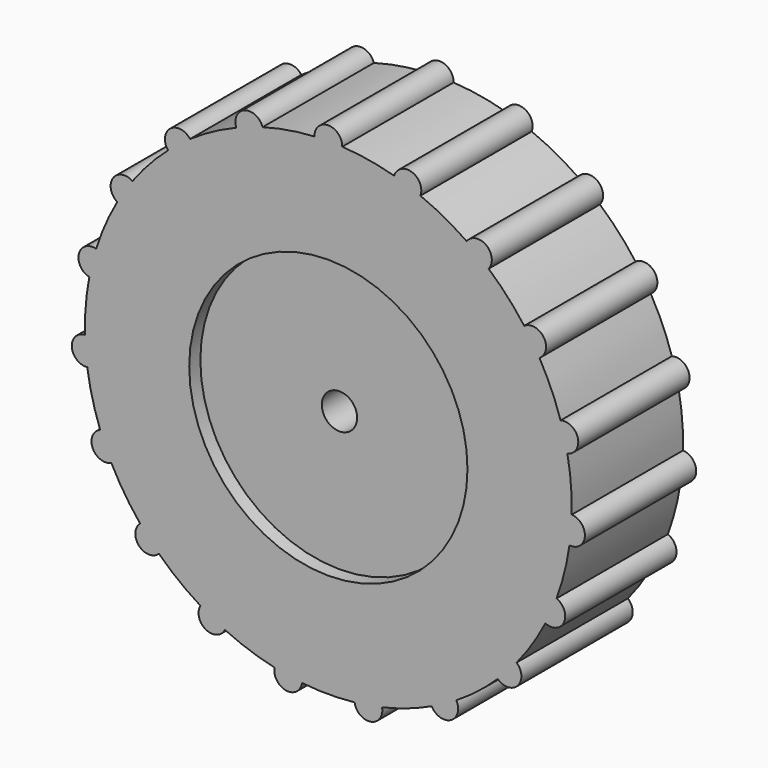
from build123d import *

# Parameters (mm, degrees)
F0_R     = 16.51
F0_R_2   = 1.6129
F1_DEPTH = 12.7
F3_R     = 12.7
F3_R_2   = 1.6129
F2_R     = 12.7
F2_R_2   = 1.6129
F4_DEPTH = 1.27
F5_DEPTH = 1.27


# Not quite as in the source:
# - the program builds the solid bodies; features that only make, move or delete a surface that nothing else refers to are left out


with BuildPart() as f1:
    # F0 (on Front) → F1 (new body)
    with BuildSketch(Plane.XZ):
        with BuildLine():
            ThreePointArc((1.2694815268, 22.1887142857), (0, 23.495), (-1.2694815268, 22.1887142857))
            ThreePointArc((-1.2694815268, 22.1887142857), (-3.658114769, 21.9218799681), (-6.0039662348, 21.3986685205))
            ThreePointArc((-6.0039662348, 21.3986685205), (-7.628814029, 22.2219760938), (-8.405361267, 20.5742685647))
            ThreePointArc((-8.405361267, 20.5742685647), (-10.5779308102, 19.5463041206), (-12.6267910938, 18.2897449866))
            ThreePointArc((-12.6267910938, 18.2897449866), (-13.6508775395, 17.5386478213), (-14.6303896913, 16.730281602))
            ThreePointArc((-14.6303896913, 16.730281602), (-16.3514639147, 15.0525829294), (-17.8813072129, 13.1988437887))
            ThreePointArc((-17.8813072129, 13.1988437887), (-18.6060249794, 12.1559228143), (-19.2699883786, 11.0733090306))
            ThreePointArc((-19.2699883786, 11.0733090306), (-20.3530621849, 8.9276808129), (-21.1981062384, 6.6776430652))
            ThreePointArc((-21.1981062384, 6.6776430652), (-21.5449209105, 5.4559149517), (-21.8213848205, 4.2163716058))
            ThreePointArc((-21.8213848205, 4.2163716058), (-22.1490903571, 1.8353259531), (-22.2177615305, -0.5671838988))
            ThreePointArc((-22.2177615305, -0.5671838988), (-22.1490903571, -1.8353259531), (-22.0080956233, -3.0974751064))
            ThreePointArc((-22.0080956233, -3.0974751064), (-21.5449209105, -5.4559149517), (-20.8297776166, -7.7505476866))
            ThreePointArc((-20.8297776166, -7.7505476866), (-20.3530621849, -8.9276808129), (-19.8098877746, -10.0756623284))
            ThreePointArc((-19.8098877746, -10.0756623284), (-18.6060249794, -12.1559228143), (-17.1845640907, -14.0940193703))
            ThreePointArc((-17.1845640907, -14.0940193703), (-16.3514639147, -15.0525829294), (-15.4649712035, -15.9619951972))
            ThreePointArc((-15.4649712035, -15.9619951972), (-13.6508775395, -17.5386478213), (-11.6771363996, -18.9101853641))
            ThreePointArc((-11.6771363996, -18.9101853641), (-10.5779308102, -19.5463041206), (-9.4441850386, -20.1185982105))
            ThreePointArc((-9.4441850386, -20.1185982105), (-7.2164457031, -21.0207881968), (-4.9043097902, -21.6771393519))
            ThreePointArc((-4.9043097902, -21.6771393519), (-3.658114769, -21.9218799681), (-2.3999748833, -22.0950389355))
            ThreePointArc((-2.3999748833, -22.0950389355), (0, -22.225), (2.3999748833, -22.0950389355))
            ThreePointArc((2.3999748833, -22.0950389355), (3.658114769, -21.9218799681), (4.9043097902, -21.6771393519))
            ThreePointArc((4.9043097902, -21.6771393519), (7.2164457031, -21.0207881968), (9.4441850386, -20.1185982105))
            ThreePointArc((9.4441850386, -20.1185982105), (10.5779308102, -19.5463041206), (11.6771363996, -18.9101853641))
            ThreePointArc((11.6771363996, -18.9101853641), (13.6508775395, -17.5386478213), (15.4649712035, -15.9619951972))
            ThreePointArc((15.4649712035, -15.9619951972), (16.3514639147, -15.0525829294), (17.1845640907, -14.0940193703))
            ThreePointArc((17.1845640907, -14.0940193703), (18.6060249794, -12.1559228143), (19.8098877746, -10.0756623284))
            ThreePointArc((19.8098877746, -10.0756623284), (20.3530621849, -8.9276808129), (20.8297776166, -7.7505476866))
            ThreePointArc((20.8297776166, -7.7505476866), (21.5449209105, -5.4559149517), (22.0080956233, -3.0974751064))
            ThreePointArc((22.0080956233, -3.0974751064), (22.1490903571, -1.8353259531), (22.2177615305, -0.5671838988))
            ThreePointArc((22.2177615305, -0.5671838988), (22.1490903571, 1.8353259531), (21.8213848205, 4.2163716058))
            ThreePointArc((21.8213848205, 4.2163716058), (21.5449209105, 5.4559149517), (21.1981062384, 6.6776430652))
            ThreePointArc((21.1981062384, 6.6776430652), (20.3530621849, 8.9276808129), (19.2699883786, 11.0733090306))
            ThreePointArc((19.2699883786, 11.0733090306), (18.6060249794, 12.1559228143), (17.8813072129, 13.1988437887))
            ThreePointArc((17.8813072129, 13.1988437887), (16.3514639147, 15.0525829294), (14.6303896913, 16.730281602))
            ThreePointArc((14.6303896913, 16.730281602), (13.6508775395, 17.5386478213), (12.6267910938, 18.2897449866))
            ThreePointArc((12.6267910938, 18.2897449866), (10.5779308102, 19.5463041206), (8.405361267, 20.5742685647))
            ThreePointArc((8.405361267, 20.5742685647), (7.628814029, 22.2219760938), (6.0039662348, 21.3986685205))
            ThreePointArc((6.0039662348, 21.3986685205), (3.658114769, 21.9218799681), (1.2694815268, 22.1887142857))
        make_face()
        Circle(F0_R, mode=Mode.SUBTRACT)
        Circle(F0_R)
        Circle(F0_R_2, mode=Mode.SUBTRACT)
        with BuildLine():
            ThreePointArc((-19.2699883786, 11.0733090306), (-18.6060249794, 12.1559228143), (-17.8813072129, 13.1988437887))
            ThreePointArc((-17.8813072129, 13.1988437887), (-19.6692264068, 12.8505469751), (-19.2699883786, 11.0733090306))
        make_face()
        with BuildLine():
            ThreePointArc((-14.6303896913, 16.730281602), (-13.6508775395, 17.5386478213), (-12.6267910938, 18.2897449866))
            ThreePointArc((-12.6267910938, 18.2897449866), (-14.4309276846, 18.5408562683), (-14.6303896913, 16.730281602))
        make_face()
        with BuildLine():
            ThreePointArc((14.6303896913, 16.730281602), (14.4309276846, 18.5408562683), (12.6267910938, 18.2897449866))
            ThreePointArc((12.6267910938, 18.2897449866), (13.6508775395, 17.5386478213), (14.6303896913, 16.730281602))
        make_face()
        with BuildLine():
            ThreePointArc((19.2699883786, 11.0733090306), (19.6692264068, 12.8505469751), (17.8813072129, 13.1988437887))
            ThreePointArc((17.8813072129, 13.1988437887), (18.6060249794, 12.1559228143), (19.2699883786, 11.0733090306))
        make_face()
        with BuildLine():
            ThreePointArc((21.8213848205, 4.2163716058), (22.7760592482, 5.7676815204), (21.1981062384, 6.6776430652))
            ThreePointArc((21.1981062384, 6.6776430652), (21.5449209105, 5.4559149517), (21.8213848205, 4.2163716058))
        make_face()
        with BuildLine():
            ThreePointArc((22.0080956233, -3.0974751064), (23.4147526632, -1.9402017219), (22.2177615305, -0.5671838988))
            ThreePointArc((22.2177615305, -0.5671838988), (22.1490903571, -1.8353259531), (22.0080956233, -3.0974751064))
        make_face()
        with BuildLine():
            ThreePointArc((-21.8213848205, 4.2163716058), (-21.5449209105, 5.4559149517), (-21.1981062384, 6.6776430652))
            ThreePointArc((-21.1981062384, 6.6776430652), (-22.7760592482, 5.7676815204), (-21.8213848205, 4.2163716058))
        make_face()
        with BuildLine():
            ThreePointArc((-22.0080956233, -3.0974751064), (-22.1490903571, -1.8353259531), (-22.2177615305, -0.5671838988))
            ThreePointArc((-22.2177615305, -0.5671838988), (-23.4147526632, -1.9402017219), (-22.0080956233, -3.0974751064))
        make_face()
        with BuildLine():
            ThreePointArc((-19.8098877746, -10.0756623284), (-20.3530621849, -8.9276808129), (-20.8297776166, -7.7505476866))
            ThreePointArc((-20.8297776166, -7.7505476866), (-21.5160943098, -9.4378340022), (-19.8098877746, -10.0756623284))
        make_face()
        with BuildLine():
            ThreePointArc((-15.4649712035, -15.9619951972), (-16.3514639147, -15.0525829294), (-17.1845640907, -14.0940193703))
            ThreePointArc((-17.1845640907, -14.0940193703), (-17.2858332813, -15.9127305253), (-15.4649712035, -15.9619951972))
        make_face()
        with BuildLine():
            ThreePointArc((-9.4441850386, -20.1185982105), (-10.5779308102, -19.5463041206), (-11.6771363996, -18.9101853641))
            ThreePointArc((-11.6771363996, -18.9101853641), (-11.1823839994, -20.6632357846), (-9.4441850386, -20.1185982105))
        make_face()
        with BuildLine():
            ThreePointArc((-2.3999748833, -22.0950389355), (-3.658114769, -21.9218799681), (-4.9043097902, -21.6771393519))
            ThreePointArc((-4.9043097902, -21.6771393519), (-3.8671498986, -23.1745588234), (-2.3999748833, -22.0950389355))
        make_face()
        with BuildLine():
            ThreePointArc((2.3999748833, -22.0950389355), (3.8671498986, -23.1745588234), (4.9043097902, -21.6771393519))
            ThreePointArc((4.9043097902, -21.6771393519), (3.658114769, -21.9218799681), (2.3999748833, -22.0950389355))
        make_face()
        with BuildLine():
            ThreePointArc((9.4441850386, -20.1185982105), (11.1823839994, -20.6632357846), (11.6771363996, -18.9101853641))
            ThreePointArc((11.6771363996, -18.9101853641), (10.5779308102, -19.5463041206), (9.4441850386, -20.1185982105))
        make_face()
        with BuildLine():
            ThreePointArc((15.4649712035, -15.9619951972), (17.2858332813, -15.9127305253), (17.1845640907, -14.0940193703))
            ThreePointArc((17.1845640907, -14.0940193703), (16.3514639147, -15.0525829294), (15.4649712035, -15.9619951972))
        make_face()
        with BuildLine():
            ThreePointArc((19.8098877746, -10.0756623284), (21.5160943098, -9.4378340022), (20.8297776166, -7.7505476866))
            ThreePointArc((20.8297776166, -7.7505476866), (20.3530621849, -8.9276808129), (19.8098877746, -10.0756623284))
        make_face()
    extrude(amount=F1_DEPTH)

    # F3 (on face) + F2 (on face) → F4 (cut)
    with BuildSketch(Plane(origin=(0, 0, 0), x_dir=(-1, 0, 0), z_dir=(0, 1, 0))):
        Circle(F3_R)
        Circle(F3_R_2, mode=Mode.SUBTRACT)
    with BuildSketch(Plane.XZ.offset(12.7)):
        Circle(F2_R)
        Circle(F2_R_2, mode=Mode.SUBTRACT)
    extrude(amount=-F4_DEPTH, dir=(0, 1, 0), mode=Mode.SUBTRACT)

    # F2 (on face) → F5 (cut)
    with BuildSketch(Plane.XZ.offset(12.7)):
        Circle(F2_R)
    extrude(amount=-F5_DEPTH, mode=Mode.SUBTRACT)


solid = f1.part
